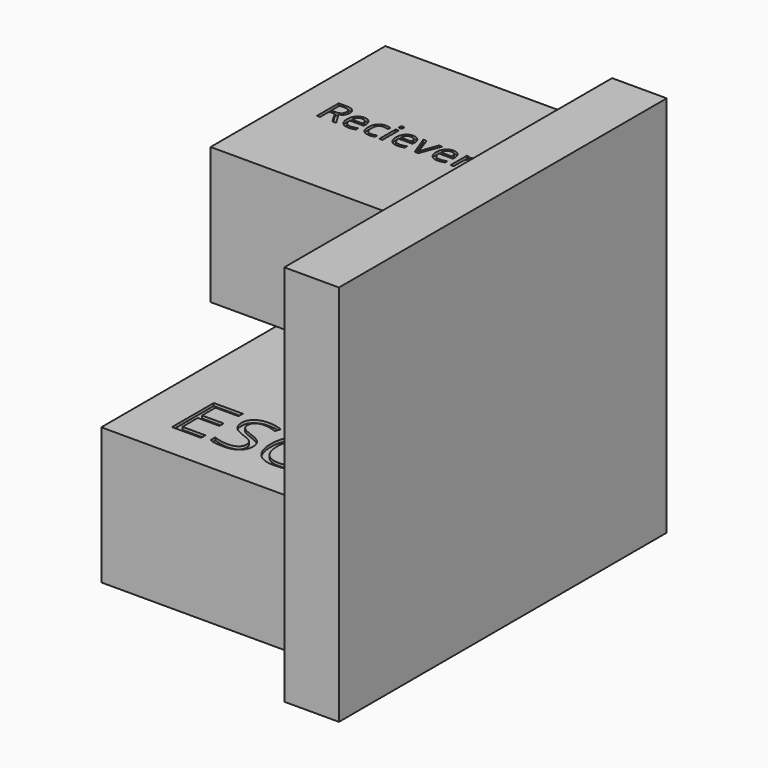
from build123d import *

# Parameters (mm, degrees)
F0_W         = 150
F0_H         = 140
F1_DEPTH     = 20
F2_W         = 80
F2_H         = 50
F3_DEPTH     = 75
F4_TEXT_SIZE = 13.8888888889
F5_TEXT_SIZE = 26.7475765819
F6_DEPTH     = 1


# Not quite as in the source:
# - Text() gives the source's letters only with a copy of the font that has no kerning and outlines rounded to 1/6400 em; it was checked with that copy


with BuildPart() as f1:
    # F0 (on Right) → F1 (new body)
    with BuildSketch(Plane.YZ):
        with Locations((75, 70)):
            Rectangle(F0_W, F0_H)
    extrude(amount=F1_DEPTH)

    # F2 (on face) → F3 (join)
    with BuildSketch(Plane(origin=(0, 0, 0), x_dir=(0, -1, 0), z_dir=(-1, 0, 0))):
        with Locations((-100, 105)):
            Rectangle(F2_W, F2_H)
        with Locations((-50, 35)):
            Rectangle(F2_W, F2_H)
    extrude(amount=F3_DEPTH)

    # F4 (on face) + F5 (on face) → F6 (cut)
    with BuildSketch(Plane.XY.offset(130)):
        with Locations((-64.6644905319, 94.1021722776)):
            Text('Reciever', F4_TEXT_SIZE, font='Open Sans', text_align=(TextAlign.LEFT, TextAlign.BOTTOM))
    with BuildSketch(Plane.XY.offset(60)):
        with Locations((-61.9145035744, 22.7290894836)):
            Text('ESC', F5_TEXT_SIZE, font='Open Sans', text_align=(TextAlign.LEFT, TextAlign.BOTTOM))
    extrude(amount=-F6_DEPTH, mode=Mode.SUBTRACT)


solid = f1.part
